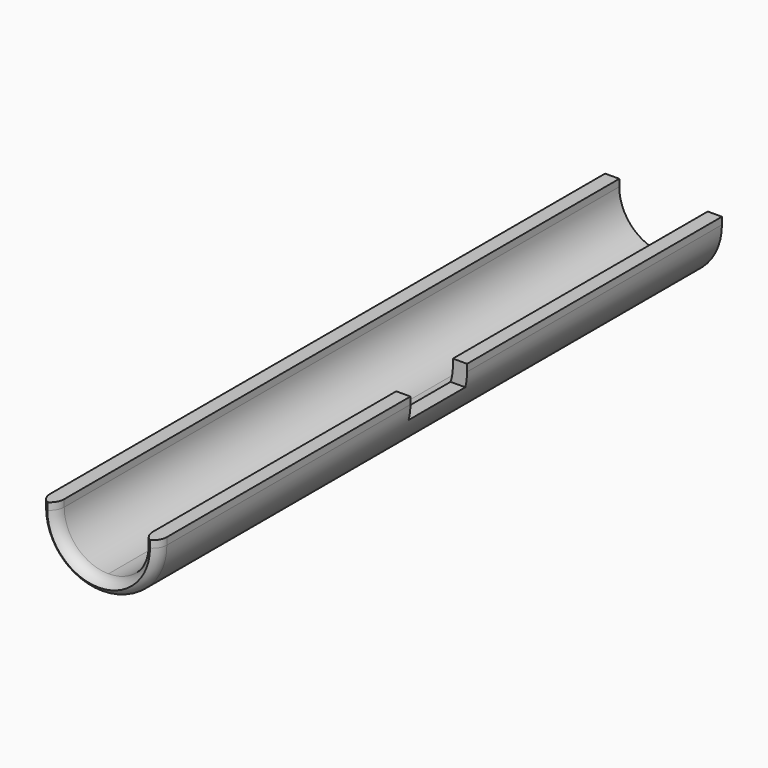
from build123d import *

# Parameters (mm, degrees)
F1_DEPTH    = 127
F2_W        = 12.7
F2_H        = 2.54
F2_H_2      = 1.27
F3_DEPTH    = 9.525
F4_T1_DEPTH = 7.62
F4_T4_ANGLE = 180
F4_T6_ANGLE = 180


# Not quite as in the source:
# - a fillet or chamfer that OpenCascade refuses, or shapes differently, is made with other operations: its cross-section is extruded or revolved along the edge and cut away or added


with BuildPart() as f1:
    # F0 (on Front) → F1 (new body)
    with BuildSketch(Plane.XZ):
        with BuildLine():
            ThreePointArc((0, -7.9375), (-5.6126600757, -5.6126600757), (-7.9375, 0))
            Line((-7.9375, 0), (-7.9375, 1.27))
            Line((-7.9375, 1.27), (-10.4775, 1.27))
            Line((-10.4775, 1.27), (-10.4775, 0))
            ThreePointArc((-10.4775, 0), (0, -10.4775), (10.4775, 0))
            Line((10.4775, 0), (10.4775, 1.27))
            Line((10.4775, 1.27), (7.9375, 1.27))
            Line((7.9375, 1.27), (7.9375, 0))
            ThreePointArc((7.9375, 0), (5.6126600757, -5.6126600757), (0, -7.9375))
        make_face()
    extrude(amount=F1_DEPTH)

    # F2 (on face) → F3 (cut)
    with BuildSketch(Plane.YZ.offset(10.4775)):
        with Locations((-63.5, -1.27)):
            Rectangle(F2_W, F2_H)
        with Locations((-63.5, 0.635)):
            Rectangle(F2_W, F2_H_2)
    extrude(amount=-F3_DEPTH, mode=Mode.SUBTRACT)

    # F4: fillet of radius 2.54 on 2 edges, made by hand

    # F4_s2 → F4_t1 (cut)
    with BuildSketch(Plane.XY):
        with BuildLine():
            ThreePointArc((-10.4775, -124.46), (-9.7335512242, -126.2560512242), (-7.9375, -127))
            Line((-7.9375, -127), (-10.4775, -127))
            Line((-10.4775, -127), (-10.4775, -124.46))
        make_face()
        with BuildLine():
            ThreePointArc((10.4775, -124.46), (9.7335512242, -126.2560512242), (7.9375, -127))
            Line((7.9375, -127), (10.4775, -127))
            Line((10.4775, -127), (10.4775, -124.46))
        make_face()
        with BuildLine():
            ThreePointArc((-7.9375, -124.46), (-8.6814487758, -126.2560512242), (-10.4775, -127))
            Line((-10.4775, -127), (-7.9375, -127))
            Line((-7.9375, -127), (-7.9375, -124.46))
        make_face()
        with BuildLine():
            ThreePointArc((10.4775, -127), (8.6814487758, -126.2560512242), (7.9375, -124.46))
            Line((7.9375, -124.46), (7.9375, -127))
            Line((7.9375, -127), (10.4775, -127))
        make_face()
    extrude(amount=F4_T1_DEPTH, mode=Mode.SUBTRACT)

    # F4_s3 → F4_t4 (revolve, cut)
    with BuildSketch(Plane.XY):
        with BuildLine():
            ThreePointArc((-7.9375, -124.46), (-8.6814487758, -126.2560512242), (-10.4775, -127))
            Line((-10.4775, -127), (-7.9375, -127))
            Line((-7.9375, -127), (-7.9375, -124.46))
        make_face()
    revolve(axis=Axis((0, -127, 0), (0, -1, 0)), revolution_arc=F4_T4_ANGLE, mode=Mode.SUBTRACT)

    # F4_s5 → F4_t6 (revolve, cut)
    with BuildSketch(Plane.XY):
        with BuildLine():
            ThreePointArc((-10.4775, -124.46), (-9.7335512242, -126.2560512242), (-7.9375, -127))
            Line((-7.9375, -127), (-10.4775, -127))
            Line((-10.4775, -127), (-10.4775, -124.46))
        make_face()
    revolve(axis=Axis((0, -127, 0), (0, -1, 0)), revolution_arc=F4_T6_ANGLE, mode=Mode.SUBTRACT)


solid = f1.part
